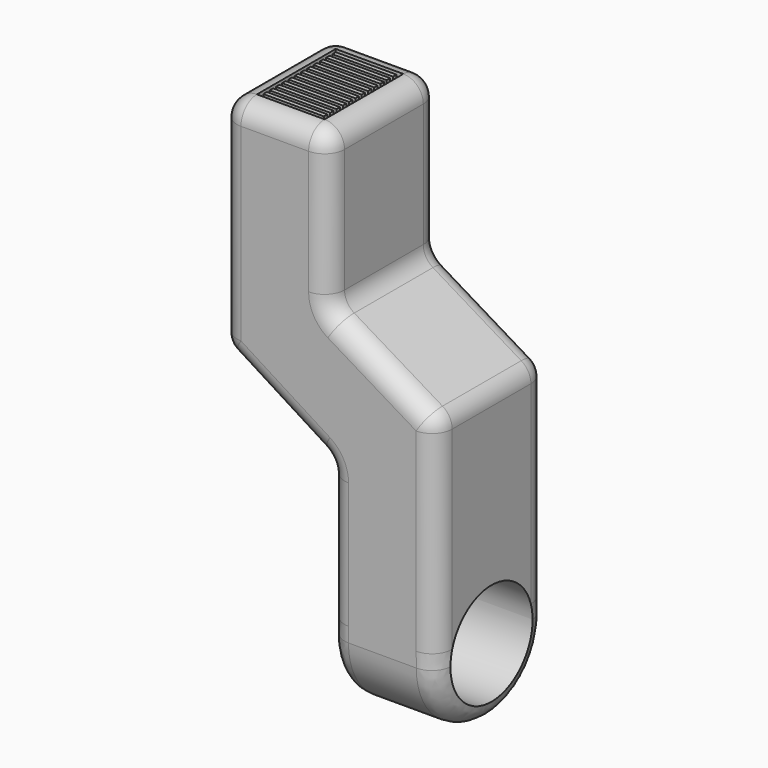
from build123d import *

# Parameters (mm, degrees)
F0_R     = 3.34
F1_DEPTH = 7
F3_DEPTH = 9
F4_DEPTH = 9.001
F5_R     = 1.3
F6_W     = 3.9447422773
F6_H     = 0.2829339355
F6_W_2   = 4.4
F6_H_2   = 6.4
F7_DEPTH = 0.5


# Not quite as in the source:
# - a feature names something its author has since deleted; it is built from what else it names


with BuildPart() as f1:
    # F0 (on Right) → F1 (new body)
    with BuildSketch(Plane.YZ):
        with BuildLine():
            Line((4.5, -14.3079506601), (4.5, 14.3079506601))
            Line((4.5, 14.3079506601), (-4.5, 14.3079506601))
            Line((-4.5, 14.3079506601), (-4.5, -14.3079506601))
            ThreePointArc((-4.5, -14.3079506601), (0, -18.8079506601), (4.5, -14.3079506601))
        make_face()
        with Locations((0, -14.3079506601)):
            Circle(F0_R, mode=Mode.SUBTRACT)
    extrude(amount=F1_DEPTH)

    # F2 (on face) → F3 (join)
    with BuildSketch(Plane.XZ.offset(4.5)):
        Polygon((0, 4.22267057), (0, 14.3079506601), (-7, 14.3079506601), (-7, 0), (0, -4.4198017567), align=None)
    extrude(amount=-F3_DEPTH)

    # F2 (on face) → F4 (cut, through all)
    with BuildSketch(Plane.XZ.offset(4.5)):
        Polygon((7, 14.3079506601), (0, 14.3079506601), (0, 4.22267057), (7, 0), align=None)
    extrude(amount=-F4_DEPTH, mode=Mode.SUBTRACT)

    # F5
    f5_edges = [f1.edges().sort_by_distance(p)[0] for p in [
        (0, -4.5, 9.265311),
        (0, 0, 4.222671),
        (0, 4.5, 9.265311),
        (0, 0, 14.307951),
        (3.5, -4.5, 2.111335),
        (-3.5, -4.5, 14.307951),
        (-7, -4.5, 7.153975),
        (-3.5, -4.5, -2.209901),
        (0, -4.5, -9.363876),
        (3.5, -4.5, -14.307951),
        (7, -4.5, -7.153975),
        (0, 4.5, -9.363876),
        (-3.5, 4.5, -2.209901),
        (-7, 4.5, 7.153975),
        (-3.5, 4.5, 14.307951),
        (3.5, 4.5, 2.111335),
        (7, 4.5, -7.153975),
        (3.5, 4.5, -14.307951),
        (-7, 0, 14.307951),
        (-7, 0, 0),
        (7, 0, 0),
        (0, 0, -4.419802),
    ]]
    fillet(f5_edges, radius=F5_R)

    # F6 (on face) → F7 (cut)
    with BuildSketch(Plane.XY.offset(14.3079506601)):
        with Locations((46.5, 2.275798656)):
            Rectangle(F6_W, F6_H)
        with Locations((46.5, 0.2357986942)):
            Rectangle(F6_W, F6_H)
        with Locations((46.5, -1.8042012677)):
            Rectangle(F6_W, F6_H)
        with Locations((46.5, 0.7457986847)):
            Rectangle(F6_W, F6_H)
        with Locations((46.5, 1.2557986751)):
            Rectangle(F6_W, F6_H)
        with Locations((46.5, -2.3142012581)):
            Rectangle(F6_W, F6_H)
        with Locations((46.5, 2.7857986465)):
            Rectangle(F6_W, F6_H)
        with Locations((46.5, -0.2742012963)):
            Rectangle(F6_W, F6_H)
        with Locations((46.5, -1.2942012772)):
            Rectangle(F6_W, F6_H)
        with Locations((46.5, 1.7657986656)):
            Rectangle(F6_W, F6_H)
        with Locations((46.5, -0.7842012867)):
            Rectangle(F6_W, F6_H)
        with Locations((46.5, -2.8242012486)):
            Rectangle(F6_W, F6_H)
        with Locations((-3.5, 0)):
            Rectangle(F6_W_2, F6_H_2)
        with Locations((-3.5, -2.8242012486)):
            Rectangle(F6_W, F6_H, mode=Mode.SUBTRACT)
        with Locations((-3.5, -2.3142012581)):
            Rectangle(F6_W, F6_H, mode=Mode.SUBTRACT)
        with Locations((-3.5, -1.8042012677)):
            Rectangle(F6_W, F6_H, mode=Mode.SUBTRACT)
        with Locations((-3.5, -1.2942012772)):
            Rectangle(F6_W, F6_H, mode=Mode.SUBTRACT)
        with Locations((-3.5, -0.7842012867)):
            Rectangle(F6_W, F6_H, mode=Mode.SUBTRACT)
        with Locations((-3.5, -0.2742012963)):
            Rectangle(F6_W, F6_H, mode=Mode.SUBTRACT)
        with Locations((-3.5, 0.2357986942)):
            Rectangle(F6_W, F6_H, mode=Mode.SUBTRACT)
        with Locations((-3.5, 0.7457986847)):
            Rectangle(F6_W, F6_H, mode=Mode.SUBTRACT)
        with Locations((-3.5, 1.2557986751)):
            Rectangle(F6_W, F6_H, mode=Mode.SUBTRACT)
        with Locations((-3.5, 1.7657986656)):
            Rectangle(F6_W, F6_H, mode=Mode.SUBTRACT)
        with Locations((-3.5, 2.275798656)):
            Rectangle(F6_W, F6_H, mode=Mode.SUBTRACT)
        with Locations((-3.5, 2.7857986465)):
            Rectangle(F6_W, F6_H, mode=Mode.SUBTRACT)
    extrude(amount=-F7_DEPTH, mode=Mode.SUBTRACT)


solid = f1.part
